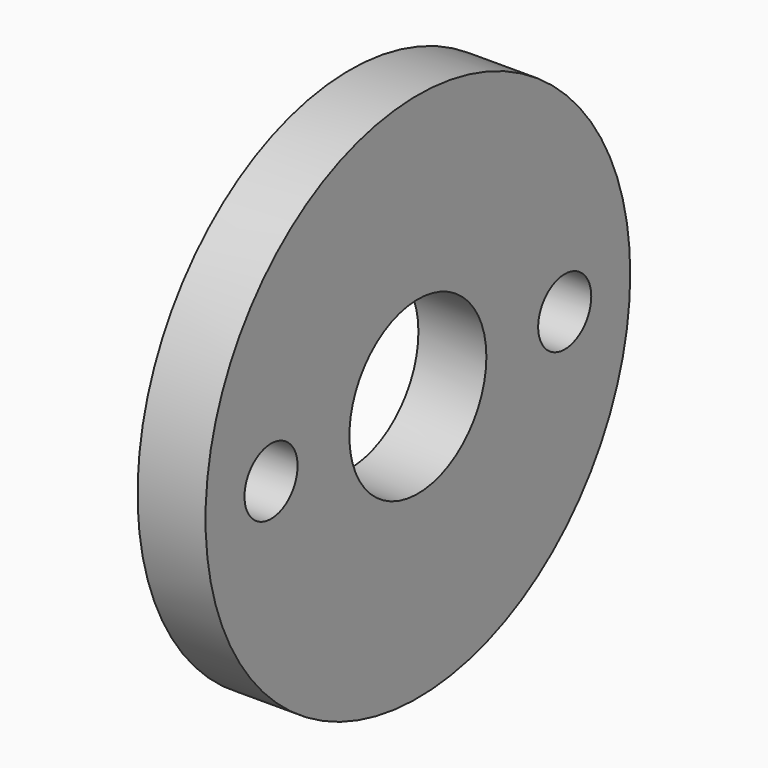
from build123d import *

# Parameters (mm, degrees)
F0_R     = 12.4
F0_R_2   = 1.55
F0_R_3   = 4
F1_DEPTH = 3.175


# Not quite as in the source:
# - a length typed as a fraction of an inch, garbled in the dataset ("3 / 203.2 mm" for 3/8 in), is restored


with BuildPart() as f1:
    # F0 (on Right) → F1 (new body)
    with BuildSketch(Plane.YZ):
        Circle(F0_R)
        with Locations((-8.575, 0)):
            Circle(F0_R_2, mode=Mode.SUBTRACT)
        Circle(F0_R_3, mode=Mode.SUBTRACT)
        with Locations((8.575, 0)):
            Circle(F0_R_2, mode=Mode.SUBTRACT)
    extrude(amount=F1_DEPTH)


solid = f1.part
